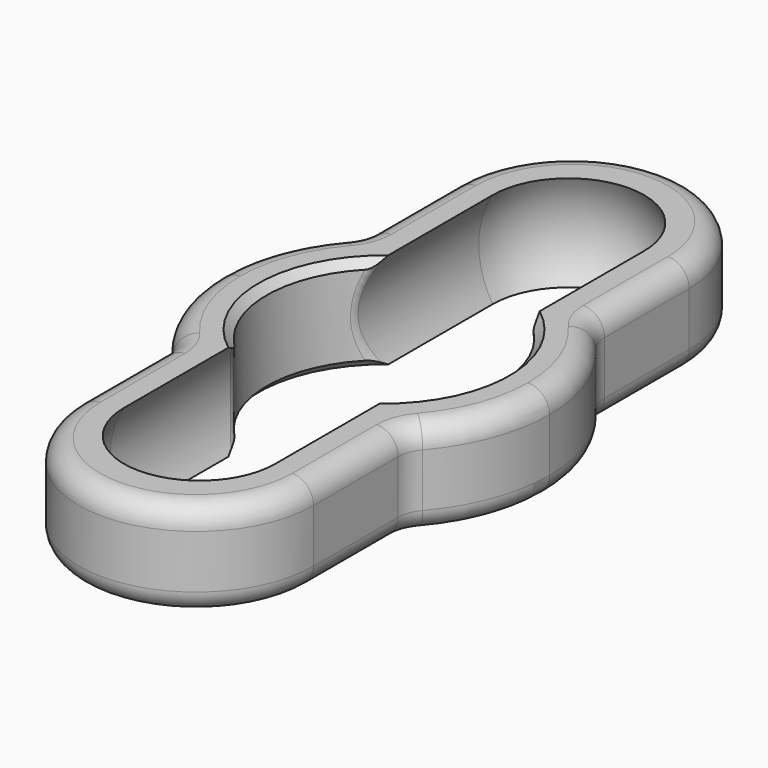
from build123d import *

# Parameters (mm, degrees)
F1_DEPTH      = 4.5
F1_DEPTH_BACK = 4.5
F2_R          = 8.4
F3_DEPTH      = 30
F4_R          = 8.4
F5_R          = 3
F7_T2_ANGLE   = 69.9434582803
F7_T4_ANGLE   = 69.9434582803
F7_T6_ANGLE   = 69.9434582803
F7_T8_ANGLE   = 69.9434582803
F8_R          = 1
F10_COUNT     = 2
F11_R         = 2


# Not quite as in the source:
# - a fillet or chamfer that OpenCascade refuses, or shapes differently, is made with other operations: its cross-section is extruded or revolved along the edge and cut away or added


with BuildPart() as f1:
    # F0 (on Top) → F1 (new body, two sides)
    with BuildSketch(Plane.XY) as f1_sk:
        with BuildLine():
            ThreePointArc((-11, 0), (0, 11), (11, 0))
            Line((11, 0), (15.5, 0))
            ThreePointArc((15.5, 0), (14.330910648, 5.9055059055), (11, 10.9201648339))
            Line((11, 10.9201648339), (11, 22))
            ThreePointArc((11, 22), (0, 33), (-11, 22))
            Line((-11, 22), (-11, 10.9201648339))
            ThreePointArc((-11, 10.9201648339), (-14.330910648, 5.9055059055), (-15.5, 0))
            Line((-15.5, 0), (-11, 0))
        make_face()
    extrude(amount=F1_DEPTH)
    extrude(f1_sk.sketch, amount=-F1_DEPTH_BACK)

    # F5
    f5_edges = [f1.edges().sort_by_distance(p)[0] for p in [
        (-11, 10.920165, 0),
        (11, 10.920165, 0),
    ]]
    fillet(f5_edges, radius=F5_R)


with BuildPart() as f3:
    # F2 (on Front) → F3 (new body)
    with BuildSketch(Plane.XZ):
        Circle(F2_R)
    extrude(amount=-F3_DEPTH)

    # F4
    f4_edges = [f3.edges().sort_by_distance(p)[0] for p in [
        (-8.4, 30, 0),
    ]]
    fillet(f4_edges, radius=F4_R)


with BuildPart() as f1_1:
    add(f1.part)

    # F6: cut F3
    add(f3.part, mode=Mode.SUBTRACT)

    # F7: chamfer of 0.75 on 4 edges, made by hand

    # F7_s1 → F7_t2 (revolve, cut)
    with BuildSketch(Plane(origin=(0, 0, 0), x_dir=(0, 0, 1), z_dir=(0.1744661978, -0.9846631636, 0))):
        Polygon((3.75, 11), (4.5, 11.75), (4.5, 11), align=None)
    revolve(axis=Axis((0, 0, 4.5), (0, 0, -1)), revolution_arc=F7_T2_ANGLE, mode=Mode.SUBTRACT)

    # F7_s3 → F7_t4 (revolve, cut)
    with BuildSketch(Plane(origin=(0, 0, 0), x_dir=(0, 0, 1), z_dir=(0.1744661978, -0.9846631636, 0))):
        Polygon((-4.5, 11.75), (-3.75, 11), (-4.5, 11), align=None)
    revolve(axis=Axis((0, 0, -4.5), (0, 0, -1)), revolution_arc=F7_T4_ANGLE, mode=Mode.SUBTRACT)

    # F7_s5 → F7_t6 (revolve, cut)
    with BuildSketch(Plane(origin=(0, 0, 0), x_dir=(0, 0, 1), z_dir=(-0.8651152041, 0.5015732087, 0))):
        Polygon((-4.5, 11.75), (-3.75, 11), (-4.5, 11), align=None)
    revolve(axis=Axis((0, 0, -4.5), (0, 0, -1)), revolution_arc=F7_T6_ANGLE, mode=Mode.SUBTRACT)

    # F7_s7 → F7_t8 (revolve, cut)
    with BuildSketch(Plane(origin=(0, 0, 0), x_dir=(0, 0, 1), z_dir=(-0.8651152041, 0.5015732087, 0))):
        Polygon((3.75, 11), (4.5, 11.75), (4.5, 11), align=None)
    revolve(axis=Axis((0, 0, 4.5), (0, 0, -1)), revolution_arc=F7_T8_ANGLE, mode=Mode.SUBTRACT)

    # F8
    f8_edges = [f1_1.edges().sort_by_distance(p)[0] for p in [
        (-8.4, 7.102112, 0),
        (8.4, 7.102112, 0),
    ]]
    fillet(f8_edges, radius=F8_R)

    # F10: F1 ×2 about axis
    f10_axis = Axis((0, 0, 12.4659836292), (0, 0, 1))


with BuildPart() as f1_2:
    add(f1_1.part)
    for i in range(1, F10_COUNT):
        add(f1_1.part.rotate(f10_axis, i * 360 / F10_COUNT))

    # F11
    f11_edges = [f1_2.edges().sort_by_distance(p)[0] for p in [
        (-11, 17.046693, 4.5),
        (11, -17.046693, -4.5),
    ]]
    fillet(f11_edges, radius=F11_R)


solid = f1_2.part
